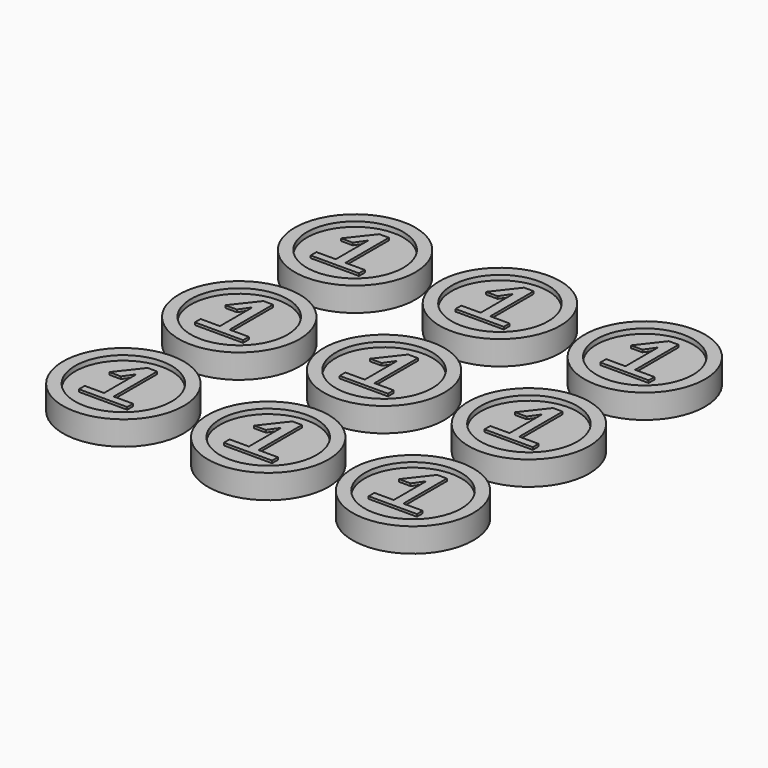
from build123d import *

# Parameters (mm, degrees)
F0_R     = 25
F0_R_2   = 20
F1_DEPTH = 5
F2_DEPTH = 3
F0_W     = 8
F0_H     = 3
F0_W_2   = 4
F3_DEPTH = 4


# Not quite as in the source:
# - a feature names something its author has since deleted; it is built from what else it names


with BuildPart() as f1:
    # F0 (on Top) → F1 (new body, symmetric)
    with BuildSketch(Plane.XY):
        Circle(F0_R)
        Circle(F0_R_2, mode=Mode.SUBTRACT)
    extrude(amount=F1_DEPTH, both=True)

    # F0 (on Top) → F2 (join, symmetric)
    with BuildSketch(Plane.XY):
        Circle(F0_R_2)
        Polygon((2, -7.5), (10, -7.5), (10, -10.5), (2, -10.5), (-2, -10.5), (-10, -10.5), (-10, -7.5), (-2, -7.5), (-2, 9.2857142857), (-5, 5), (-9.7841983661, 5), (-2, 15), (2, 15), align=None, mode=Mode.SUBTRACT)
    extrude(amount=F2_DEPTH, both=True)

    # F0 (on Top) → F3 (join, symmetric)
    with BuildSketch(Plane.XY):
        with Locations((-6, -9)):
            Rectangle(F0_W, F0_H)
        with Locations((0, -9)):
            Rectangle(F0_W_2, F0_H)
        with Locations((6, -9)):
            Rectangle(F0_W, F0_H)
        Polygon((-5, 5), (-2, 9.2857142857), (-2, 15), (-9.7841983661, 5), align=None)
        Polygon((-2, -7.5), (2, -7.5), (2, 15), (-2, 9.2857142857), align=None)
        Polygon((-2, 9.2857142857), (2, 15), (-2, 15), align=None)
    extrude(amount=F3_DEPTH, both=True)


with BuildPart() as f4_1:
    # F4: copy of F1
    add(f1.part.moved(Location((60, 0, 0))))


with BuildPart() as f5_1:
    # F5: copy of F1
    add(f1.part.moved(Location((-60, 0, 0))))


with BuildPart() as f6_1:
    # F6: copy of F1
    add(f1.part.moved(Location((-60, 60, 0))))


with BuildPart() as f7_1:
    # F7: copy of F1
    add(f1.part.moved(Location((0, 60, 0))))


with BuildPart() as f8_1:
    # F8: copy of F1
    add(f1.part.moved(Location((60, 60, 0))))


with BuildPart() as f9_1:
    # F9: copy of F1
    add(f1.part.moved(Location((60, -60, 0))))


with BuildPart() as f10_1:
    # F10: copy of F1
    add(f1.part.moved(Location((0, -60, 0))))


with BuildPart() as f11_1:
    # F11: copy of F1
    add(f1.part.moved(Location((-60, -60, 0))))


solid = Compound([f1.part, f4_1.part, f5_1.part, f6_1.part, f7_1.part, f8_1.part, f9_1.part, f10_1.part, f11_1.part])
